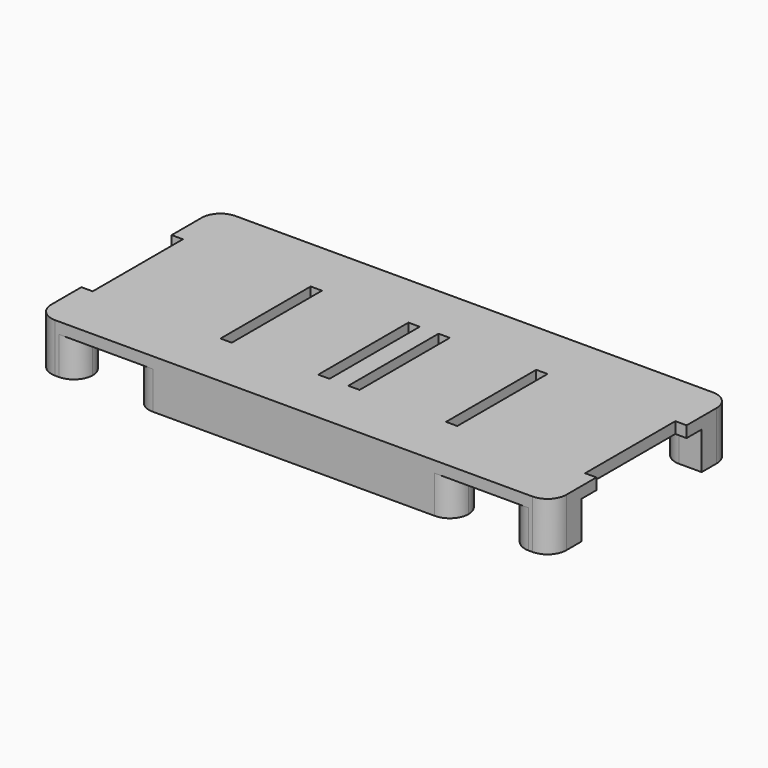
from build123d import *

# Parameters (mm, degrees)
F0_W     = 150
F0_H     = 60
F1_DEPTH = 3
F2_W     = 3
F2_H     = 30
F3_DEPTH = 25
F4_W     = 6.5
F4_H     = 60
F5_DEPTH = 25
F6_W     = 85
F6_H     = 10
F6_W_2   = 11
F7_DEPTH = 10
F8_R     = 4.99999


# Not quite as in the source:
# - a fillet or chamfer is up to 0.001 mm smaller than in the source, because OpenCascade refuses the exact size


with BuildPart() as f1:
    # F0 (on Top) → F1 (new body)
    with BuildSketch(Plane.XY):
        Rectangle(F0_W, F0_H)
    extrude(amount=F1_DEPTH)

    # F2 (on Top) → F3 (cut)
    with BuildSketch(Plane.XY):
        with Locations((-4, 0)):
            Rectangle(F2_W, F2_H)
        with Locations((4, 0)):
            Rectangle(F2_W, F2_H)
        with Locations((67, 0)):
            Rectangle(F2_W, F2_H)
        with Locations((-67, 0)):
            Rectangle(F2_W, F2_H)
        with Locations((-30, 0)):
            Rectangle(F2_W, F2_H)
        with Locations((30, 0)):
            Rectangle(F2_W, F2_H)
    extrude(amount=F3_DEPTH, mode=Mode.SUBTRACT)

    # F4 (on Top) → F5 (cut)
    with BuildSketch(Plane.XY):
        with Locations((71.75, 0)):
            Rectangle(F4_W, F4_H)
        with Locations((-71.75, 0)):
            Rectangle(F4_W, F4_H)
    extrude(amount=F5_DEPTH, mode=Mode.SUBTRACT)

    # F6 (on Top) → F7 (join)
    with BuildSketch(Plane.XY):
        with Locations((0, 25)):
            Rectangle(F6_W, F6_H)
        with Locations((0, -25)):
            Rectangle(F6_W, F6_H)
        with Locations((63, 25)):
            Rectangle(F6_W_2, F6_H)
        with Locations((63, -25)):
            Rectangle(F6_W_2, F6_H)
        with Locations((-63, -25)):
            Rectangle(F6_W_2, F6_H)
        with Locations((-63, 25)):
            Rectangle(F6_W_2, F6_H)
    extrude(amount=-F7_DEPTH)

    # F8 (radius 5 in the source; OpenCascade refuses exactly that, so slightly less here)
    f8_edges = [f1.edges().sort_by_distance(p)[0] for p in [
        (-68.5, -30, -3.5),
        (-68.5, 30, -3.5),
        (68.5, 30, -3.5),
        (68.5, -30, -3.5),
        (42.5, 30, -5),
        (42.5, 20, -5),
        (42.5, -20, -5),
        (42.5, -30, -5),
        (57.5, 30, -5),
        (57.5, 20, -5),
        (57.5, -20, -5),
        (57.5, -30, -5),
        (-42.5, 30, -5),
        (-42.5, 20, -5),
        (-42.5, -20, -5),
        (-42.5, -30, -5),
        (-57.5, 30, -5),
        (-57.5, 20, -5),
        (-57.5, -20, -5),
        (-57.5, -30, -5),
    ]]
    fillet(f8_edges, radius=F8_R)


solid = f1.part
